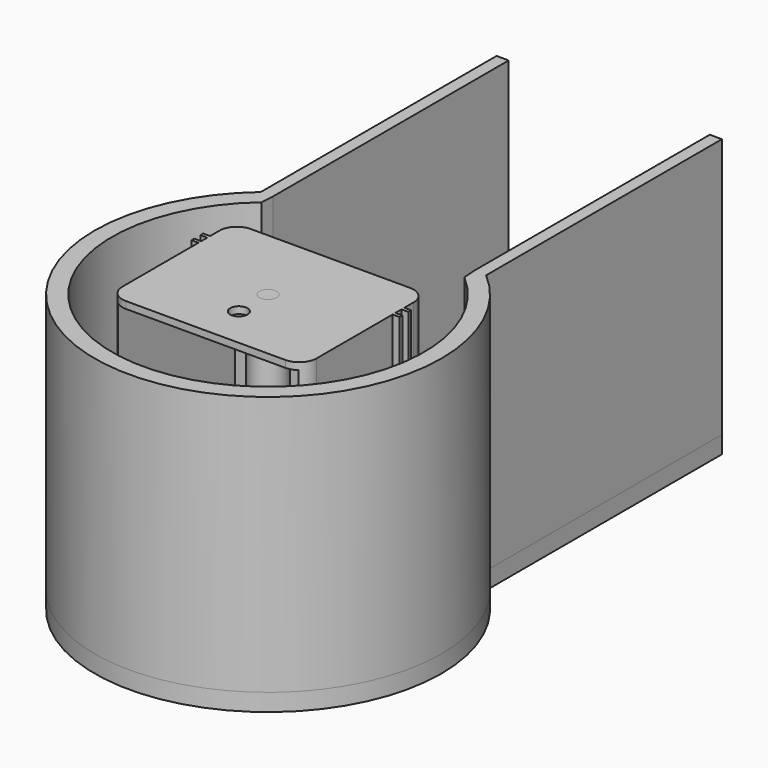
from build123d import *

# Parameters (mm, degrees)
F1_DEPTH     = 80
F3_DEPTH     = 5
F4_R         = 5
F5_DEPTH     = 80
F7_R         = 25
F8_DEPTH     = 7
F10_DEPTH    = 6
F6_R         = 5
F6_R_2       = 1.5
F11_DEPTH    = 2
F12_R        = 2.5
F12_W        = 2
F12_H        = 1
F13_DEPTH    = 80
F14_T        = 2
F14_T3_DEPTH = 84
F15_T1_DEPTH = 105
F16_R        = 2.5
F17_DEPTH    = 80
F18_R        = 10
F19_DEPTH    = 20


# Not quite as in the source:
# - a fillet or chamfer that OpenCascade refuses, or shapes differently, is made with other operations: its cross-section is extruded or revolved along the edge and cut away or added
# - a shell that OpenCascade refuses in one call is made with other operations: the cavity is built on its own and cut out


with BuildPart() as f1:
    # F0 (on Top) → F1 (new body)
    with BuildSketch(Plane.XY):
        with BuildLine():
            Line((-32.5, 122.9967103839), (-32.5, 37.9967103839))
            ThreePointArc((-32.5, 37.9967103839), (0, -50), (32.5, 37.9967103839))
            Line((32.5, 37.9967103839), (32.5, 122.9967103839))
            Line((32.5, 122.9967103839), (29, 122.9967103839))
            Line((29, 122.9967103839), (29, 37.9967103839))
            Line((29, 37.9967103839), (29.25, 34.1970393455))
            ThreePointArc((29.25, 34.1970393455), (0, -45), (-29.25, 34.1970393455))
            Line((-29.25, 34.1970393455), (-29, 37.9967103839))
            Line((-29, 37.9967103839), (-29, 122.9967103839))
            Line((-29, 122.9967103839), (-32.5, 122.9967103839))
        make_face()
    extrude(amount=F1_DEPTH)


with BuildPart() as f3:
    # F2 (on Top) → F3 (new body)
    with BuildSketch(Plane.XY):
        with BuildLine():
            Line((-32.5, 122.9967103839), (-32.5, 37.9967103839))
            ThreePointArc((-32.5, 37.9967103839), (0, -50), (32.5, 37.9967103839))
            Line((32.5, 37.9967103839), (32.5, 122.9967103839))
            Line((32.5, 122.9967103839), (-32.5, 122.9967103839))
        make_face()
    extrude(amount=F3_DEPTH)


with BuildPart() as f5:
    # F4 (on Top) → F5 (new body)
    with BuildSketch(Plane.XY):
        Circle(F4_R)
    extrude(amount=F5_DEPTH)


with BuildPart() as f8:
    # F7 (on Top) → F8 (new body)
    with BuildSketch(Plane.XY):
        Circle(F7_R)
    extrude(amount=F8_DEPTH)


with BuildPart() as f10:
    # F9 (on Top) → F10 (new body)
    with BuildSketch(Plane.XY):
        with BuildLine():
            Line((4.8166118904, 5.0793946389), (2.5867517761, 66.8409752222))
            ThreePointArc((2.5867517761, 66.8409752222), (0, 72.6986680031), (-2.5867517761, 66.8409752222))
            Line((-2.5867517761, 66.8409752222), (-4.8166118904, 5.0793946389))
            ThreePointArc((-4.8166118904, 5.0793946389), (0, -7), (4.8166118904, 5.0793946389))
        make_face()
        with BuildLine():
            ThreePointArc((4.9869817475, 0.3605732245), (4.996744377, 0.1804040778), (5, 0))
            ThreePointArc((5, 0), (0, -5), (-5, 0))
            ThreePointArc((-5, 0), (-4.996744377, 0.1804040778), (-4.9869817475, 0.3605732245))
            ThreePointArc((-4.9869817475, 0.3605732245), (0, 5), (4.9869817475, 0.3605732245))
        make_face(mode=Mode.SUBTRACT)
        with BuildLine():
            ThreePointArc((0, 66.6986680031), (-1.767766953, 70.966434956), (2.5, 69.1986680031))
            ThreePointArc((2.5, 69.1986680031), (1.767766953, 67.4309010501), (0, 66.6986680031))
        make_face(mode=Mode.SUBTRACT)
    extrude(amount=F10_DEPTH)


with BuildPart() as f11:
    # F6 (on Top) → F11 (new body)
    with BuildSketch(Plane.XY):
        with BuildLine():
            ThreePointArc((-3.6129275124, 9.3245243734), (-5.6511381542, -8.2501295482), (10, 0))
            ThreePointArc((10, 0), (8.2501295482, 5.6511381542), (3.6129275124, 9.3245243734))
            ThreePointArc((3.6129275124, 9.3245243734), (0, 10), (-3.6129275124, 9.3245243734))
        make_face()
        Circle(F6_R, mode=Mode.SUBTRACT)
        with BuildLine():
            ThreePointArc((-3.6129275124, 9.3245243734), (0, 10), (3.6129275124, 9.3245243734))
            Line((3.6129275124, 9.3245243734), (2.7659637974, 14.7827281256))
            ThreePointArc((2.7659637974, 14.7827281256), (0, 13.4273596257), (-2.7659637974, 14.7827281256))
            Line((-2.7659637974, 14.7827281256), (-3.6129275124, 9.3245243734))
        make_face()
        with BuildLine():
            ThreePointArc((-2.7659637974, 14.7827281256), (0, 13.4273596257), (2.7659637974, 14.7827281256))
            ThreePointArc((2.7659637974, 14.7827281256), (3.3114100691, 15.7939738333), (3.5, 16.9273596257))
            ThreePointArc((3.5, 16.9273596257), (-1.1333857924, 20.2387696948), (-2.7659637974, 14.7827281256))
        make_face()
        with Locations((0, 16.9273596257)):
            Circle(F6_R_2, mode=Mode.SUBTRACT)
    extrude(amount=F11_DEPTH)


with BuildPart() as f13:
    # F12 (on Top) → F13 (new body)
    with BuildSketch(Plane.XY):
        Polygon((28, 22.5), (-28, 22.5), (-28, 14.1049482152), (-28, 13.1049482152), (-28, 10.9004797414), (-28, 9.9004797414), (-28, -22.5), (28, -22.5), (28, 9.9004797414), (28, 10.9004797414), (28, 13.1049482152), (28, 14.1049482152), align=None)
        with Locations((0, -10.5241974816)):
            Circle(F12_R, mode=Mode.SUBTRACT)
        with Locations((-29, 13.6049482152)):
            Rectangle(F12_W, F12_H)
        with Locations((-29, 10.4004797414)):
            Rectangle(F12_W, F12_H)
        with Locations((29, 13.6049482152)):
            Rectangle(F12_W, F12_H)
        with Locations((29, 10.4004797414)):
            Rectangle(F12_W, F12_H)
    extrude(amount=F13_DEPTH)

    # F14: shell of thickness 2, made by hand


with BuildPart() as f14_core1:
    # F14_t2: copy of F13
    add(f13.part)

    # the walls: a layer under each face that stays
    f14_faces = [f14_core1.faces().sort_by_distance(p)[0] for p in [
        (0, 22.5, 40),
        (-28, 18.3024741076, 40),
        (-29, 14.1049482152, 40),
        (-30, 13.6049482152, 40),
        (-29, 13.1049482152, 40),
        (-28, 12.0027139783, 40),
        (-29, 10.9004797414, 40),
        (-30, 10.4004797414, 40),
        (-29, 9.9004797414, 40),
        (-28, -6.2997601293, 40),
        (28, -6.2997601293, 40),
        (29, 9.9004797414, 40),
        (30, 10.4004797414, 40),
        (29, 10.9004797414, 40),
        (28, 12.0027139783, 40),
        (29, 13.1049482152, 40),
        (30, 13.6049482152, 40),
        (29, 14.1049482152, 40),
        (28, 18.3024741076, 40),
        (0, 0, 0),
        (0, 0, 80),
    ]]
    thicken(f14_faces, amount=-F14_T, mode=Mode.SUBTRACT)

    # F14_s4 → F14_t3 (cut)
    with BuildSketch(Plane.XY.offset(-2)):
        Polygon((-28.02, 14.1249482152), (-26, 14.1049482152), (-26, 12.1049482152), (-28, 12.1049482152), align=None)
        Polygon((-28.02, 13.0849482152), (-28, 15.1049482152), (-26, 15.1049482152), (-26, 13.1049482152), align=None)
        Polygon((-28.02, 10.9204797414), (-26, 10.9004797414), (-26, 8.9004797414), (-28, 8.9004797414), align=None)
        Polygon((-28.02, 9.8804797414), (-28, 11.9004797414), (-26, 11.9004797414), (-26, 9.9004797414), align=None)
        Polygon((28.02, 9.8804797414), (26, 9.9004797414), (26, 11.9004797414), (28, 11.9004797414), align=None)
        Polygon((28.02, 10.9204797414), (28, 8.9004797414), (26, 8.9004797414), (26, 10.9004797414), align=None)
        Polygon((28.02, 13.0849482152), (26, 13.1049482152), (26, 15.1049482152), (28, 15.1049482152), align=None)
        Polygon((28.02, 14.1249482152), (28, 12.1049482152), (26, 12.1049482152), (26, 14.1049482152), align=None)
    extrude(amount=F14_T3_DEPTH, mode=Mode.SUBTRACT)


with BuildPart() as f13_1:
    add(f13.part)

    # what is left inside the walls is the cavity
    f14_cavity = [f14_core1.part.solids().sort_by_distance(p)[0] for p in [
        (0, 20.48, 52.666667),
    ]]
    add(f14_cavity, mode=Mode.SUBTRACT)

    # F15: fillet of radius 5 on 4 edges, made by hand

    # F15_s2 → F15_t1 (cut)
    with BuildSketch(Plane.XY.offset(-12.5)):
        with BuildLine():
            ThreePointArc((-23, 22.5), (-26.5355339059, 21.0355339059), (-28, 17.5))
            Line((-28, 17.5), (-28, 22.5))
            Line((-28, 22.5), (-23, 22.5))
        make_face()
        with BuildLine():
            ThreePointArc((23, 22.5), (26.5355339059, 21.0355339059), (28, 17.5))
            Line((28, 17.5), (28, 22.5))
            Line((28, 22.5), (23, 22.5))
        make_face()
        with BuildLine():
            ThreePointArc((23, -22.5), (26.5355339059, -21.0355339059), (28, -17.5))
            Line((28, -17.5), (28, -22.5))
            Line((28, -22.5), (23, -22.5))
        make_face()
        with BuildLine():
            ThreePointArc((-28, -17.5), (-26.5355339059, -21.0355339059), (-23, -22.5))
            Line((-23, -22.5), (-28, -22.5))
            Line((-28, -22.5), (-28, -17.5))
        make_face()
    extrude(amount=F15_T1_DEPTH, mode=Mode.SUBTRACT)


with BuildPart() as f17:
    # F16 (on Top) → F17 (new body)
    with BuildSketch(Plane.XY):
        Circle(F16_R)
    extrude(amount=F17_DEPTH)


with BuildPart() as f19:
    # F18 (on Top) → F19 (new body)
    with BuildSketch(Plane.XY):
        Circle(F18_R)
    extrude(amount=F19_DEPTH)


solid = Compound([f1.part, f3.part, f5.part, f8.part, f10.part, f11.part, f13_1.part, f17.part, f19.part])
